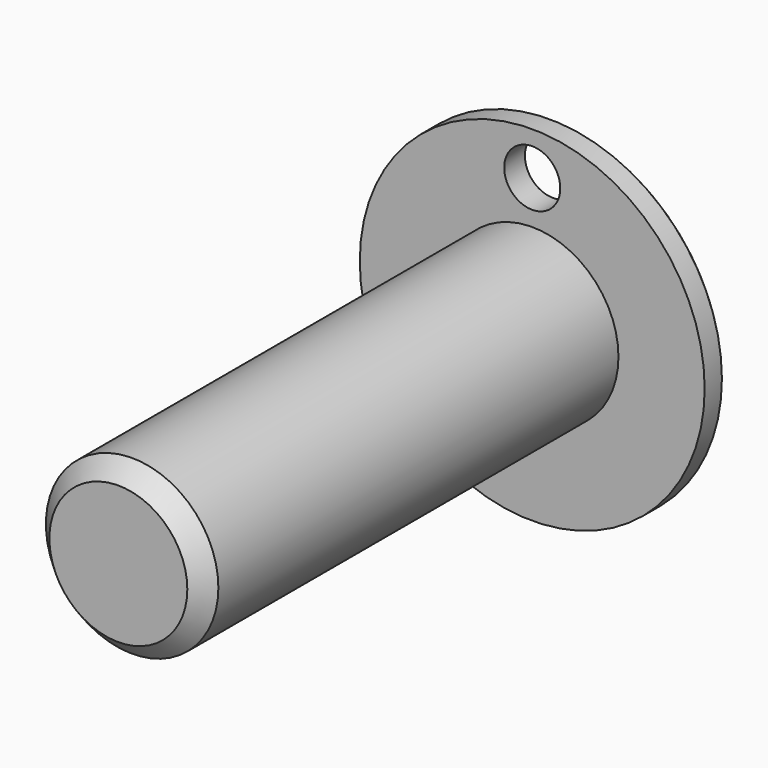
from build123d import *

# Parameters (mm, degrees)
F0_R     = 10
F1_DEPTH = 60
F2_R     = 20
F2_R_2   = 10
F3_DEPTH = 3
F4_SIZE  = 2
F6_D     = 6.5
F7_SIZE  = 0.5


with BuildPart() as f1:
    # F0 (on Front) → F1 (new body)
    with BuildSketch(Plane.XZ):
        Circle(F0_R)
    extrude(amount=F1_DEPTH)

    # F2 (on face) → F3 (join)
    with BuildSketch(Plane(origin=(0, 0, 0), x_dir=(-1, 0, 0), z_dir=(0, 1, 0))):
        Circle(F2_R)
        Circle(F2_R_2, mode=Mode.SUBTRACT)
        Circle(F2_R_2)
    extrude(amount=F3_DEPTH)

    # F4
    f4_edges = [f1.edges().sort_by_distance(p)[0] for p in [
        (-10, -60, 0),
    ]]
    chamfer(f4_edges, length=F4_SIZE)

    # F6 (through all)
    with Locations(Plane(origin=(0, 3, 0), x_dir=(-1, 0, 0), z_dir=(0, 1, 0))):
        with Locations((0, 15)):
            Hole(F6_D / 2)

    # F7
    f7_edges = [f1.edges().sort_by_distance(p)[0] for p in [
        (20, 3, 0),
    ]]
    chamfer(f7_edges, length=F7_SIZE)


solid = f1.part
